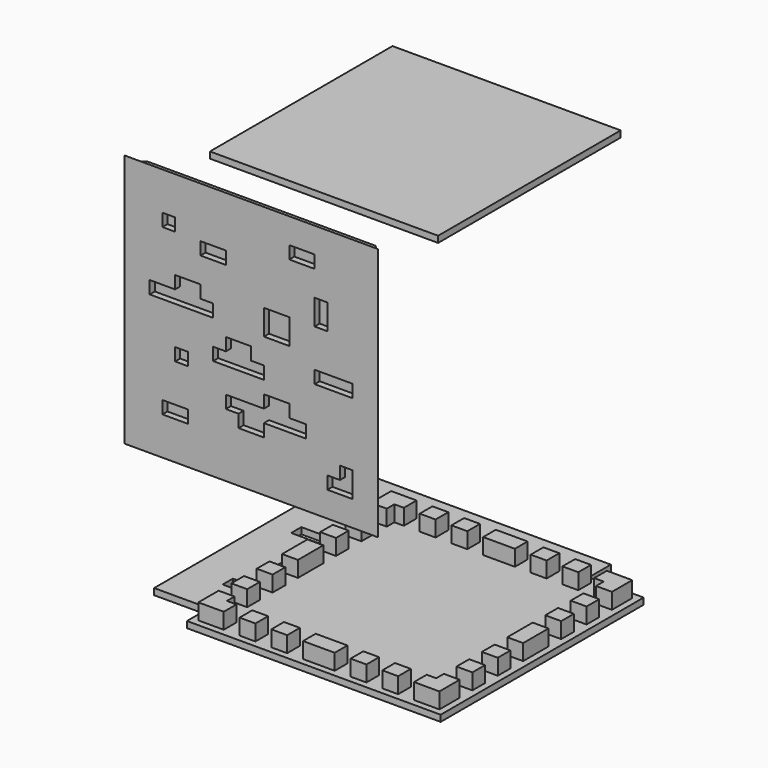
from build123d import *

# Parameters (mm, degrees)
F0_W      = 80
F0_H      = 80
F0_W_2    = 8
F0_H_2    = 4
F0_W_3    = 4
F0_W_4    = 12
F0_H_3    = 8
F1_DEPTH  = 2
F2_W      = 80
F2_H      = 80
F3_DEPTH  = 2
F4_W      = 76
F4_H      = 76
F4_W_2    = 66
F4_H_2    = 66
F5_DEPTH  = 5
F6_W      = 5
F6_H      = 5
F7_DEPTH  = 5
F8_W      = 80
F8_H      = 80
F8_W_2    = 8
F8_H_2    = 4
F8_W_3    = 4
F8_W_4    = 12
F8_H_3    = 8
F9_DEPTH  = 2
F13_DEPTH = 80
F15_DEPTH = 80
F17_DEPTH = 5
F18_W     = 12
F18_H     = 4
F18_W_2   = 8
F18_W_3   = 4
F18_H_2   = 8
F18_W_4   = 1.9
F18_H_3   = 2.2186623164
F19_DEPTH = 2
F21_DEPTH = 73
F22_DEPTH = 5
F24_W     = 71.95
F24_H     = 71.95
F25_DEPTH = 2


with BuildPart() as f1:
    # F0 (on Top) → F1 (new body)
    with BuildSketch(Plane.XY):
        with Locations((-17.2806037962, 8.6768372357)):
            Rectangle(F0_W, F0_H)
        with Locations((-41.2806037962, -17.3231627643)):
            Rectangle(F0_W_2, F0_H_2, mode=Mode.SUBTRACT)
        with Locations((-39.2806037962, -1.3231627643)):
            Rectangle(F0_W_3, F0_H_2, mode=Mode.SUBTRACT)
        Polygon((-25.2806037962, 4.6768372357), (-25.2806037962, 8.6768372357), (-17.2806037962, 8.6768372357), (-17.2806037962, 4.6768372357), (-13.2806037962, 4.6768372357), (-13.2806037962, 0.6768372357), (-29.2806037962, 0.6768372357), (-29.2806037962, 4.6768372357), align=None, mode=Mode.SUBTRACT)
        Polygon((14.7193962038, -23.3231627643), (6.7193962038, -23.3231627643), (6.7193962038, -19.3231627643), (10.7193962038, -19.3231627643), (10.7193962038, -15.3231627643), (14.7193962038, -15.3231627643), (14.7193962038, -19.3231627643), align=None, mode=Mode.SUBTRACT)
        Polygon((-13.2806037962, -7.3231627643), (-13.2806037962, -3.3231627643), (-5.2806037962, -3.3231627643), (-5.2806037962, -7.3231627643), (0, -7.3231627643), (0, -11.3231627643), (-13.2806037962, -11.3231627643), (-13.2806037962, -15.3231627643), (-21.2806037962, -15.3231627643), (-21.2806037962, -11.3231627643), (-25.2806037962, -11.3231627643), (-25.2806037962, -7.3231627643), align=None, mode=Mode.SUBTRACT)
        with Locations((8.7193962038, 6.6768372357)):
            Rectangle(F0_W_4, F0_H_2, mode=Mode.SUBTRACT)
        Polygon((-41.2806037962, 16.6768372357), (-41.2806037962, 20.6768372357), (-33.2806037962, 20.6768372357), (-33.2806037962, 16.6768372357), (-29.2806037962, 16.6768372357), (-29.2806037962, 12.6768372357), (-49.2806037962, 12.6768372357), (-49.2806037962, 16.6768372357), align=None, mode=Mode.SUBTRACT)
        with Locations((-43.2806037962, 34.6768372357)):
            Rectangle(F0_W_3, F0_H_2, mode=Mode.SUBTRACT)
        with Locations((-29.2806037962, 30.6768372357)):
            Rectangle(F0_W_2, F0_H_2, mode=Mode.SUBTRACT)
        with Locations((-9.2806037962, 16.6768372357)):
            Rectangle(F0_W_2, F0_H_3, mode=Mode.SUBTRACT)
        with Locations((4.7193962038, 24.6768372357)):
            Rectangle(F0_W_3, F0_H_3, mode=Mode.SUBTRACT)
        with Locations((-1.2806037962, 38.6768372357)):
            Rectangle(F0_W_2, F0_H_2, mode=Mode.SUBTRACT)
    extrude(amount=F1_DEPTH)


with BuildPart() as f3:
    # F2 (on Top) → F3 (new body)
    with BuildSketch(Plane.XY):
        Rectangle(F2_W, F2_H)
    extrude(amount=F3_DEPTH)

    # F4 (on face) → F5 (join)
    with BuildSketch(Plane.XY.offset(2)):
        Rectangle(F4_W, F4_H)
        Rectangle(F4_W_2, F4_H_2, mode=Mode.SUBTRACT)
    extrude(amount=F5_DEPTH)

    # F6 (on face) → F7 (cut)
    with BuildSketch(Plane.XY.offset(7)):
        with Locations((-35.5, -27.5)):
            Rectangle(F6_W, F6_H)
        with Locations((-35.5, -17.5)):
            Rectangle(F6_W, F6_H)
        with Locations((-35.5, -7.5)):
            Rectangle(F6_W, F6_H)
        with Locations((-35.5, 27.5)):
            Rectangle(F6_W, F6_H)
        with Locations((-35.5, 17.5)):
            Rectangle(F6_W, F6_H)
        with Locations((-35.5, 7.5)):
            Rectangle(F6_W, F6_H)
        with Locations((35.5, -27.5)):
            Rectangle(F6_W, F6_H)
        with Locations((35.5, -17.5)):
            Rectangle(F6_W, F6_H)
        with Locations((35.5, -7.5)):
            Rectangle(F6_W, F6_H)
        with Locations((35.5, 27.5)):
            Rectangle(F6_W, F6_H)
        with Locations((35.5, 17.5)):
            Rectangle(F6_W, F6_H)
        with Locations((35.5, 7.5)):
            Rectangle(F6_W, F6_H)
        with Locations((-27.5, 35.5)):
            Rectangle(F6_W, F6_H)
        with Locations((-17.5, 35.5)):
            Rectangle(F6_W, F6_H)
        with Locations((27.5, 35.5)):
            Rectangle(F6_W, F6_H)
        with Locations((17.5, 35.5)):
            Rectangle(F6_W, F6_H)
        with Locations((7.5, 35.5)):
            Rectangle(F6_W, F6_H)
        with Locations((-7.5, 35.5)):
            Rectangle(F6_W, F6_H)
        with Locations((-27.5, -35.5)):
            Rectangle(F6_W, F6_H)
        with Locations((-17.5, -35.5)):
            Rectangle(F6_W, F6_H)
        with Locations((-7.5, -35.5)):
            Rectangle(F6_W, F6_H)
        with Locations((27.5, -35.5)):
            Rectangle(F6_W, F6_H)
        with Locations((17.5, -35.5)):
            Rectangle(F6_W, F6_H)
        with Locations((7.5, -35.5)):
            Rectangle(F6_W, F6_H)
    extrude(amount=-F7_DEPTH, mode=Mode.SUBTRACT)


with BuildPart() as f9:
    # F8 (on Front) → F9 (new body)
    with BuildSketch(Plane.XZ):
        with Locations((-50.1320821094, 59.4921786048)):
            Rectangle(F8_W, F8_H)
        with Locations((-74.1320821094, 33.4921786048)):
            Rectangle(F8_W_2, F8_H_2, mode=Mode.SUBTRACT)
        with Locations((-72.1320821094, 49.4921786048)):
            Rectangle(F8_W_3, F8_H_2, mode=Mode.SUBTRACT)
        Polygon((-58.1320821094, 55.4921786048), (-58.1320821094, 59.4921786048), (-50.1320821094, 59.4921786048), (-50.1320821094, 55.4921786048), (-46.1320821094, 55.4921786048), (-46.1320821094, 51.4921786048), (-62.1320821094, 51.4921786048), (-62.1320821094, 55.4921786048), align=None, mode=Mode.SUBTRACT)
        Polygon((-18.1320821094, 27.4921786048), (-26.1320821094, 27.4921786048), (-26.1320821094, 31.4921786048), (-22.1320821094, 31.4921786048), (-22.1320821094, 35.4921786048), (-18.1320821094, 35.4921786048), (-18.1320821094, 31.4921786048), align=None, mode=Mode.SUBTRACT)
        Polygon((-46.1320821094, 43.4921786048), (-46.1320821094, 47.4921786048), (-38.1320821094, 47.4921786048), (-38.1320821094, 43.4921786048), (-32.8514783131, 43.4921786048), (-32.8514783131, 39.4921786048), (-46.1320821094, 39.4921786048), (-46.1320821094, 35.4921786048), (-54.1320821094, 35.4921786048), (-54.1320821094, 39.4921786048), (-58.1320821094, 39.4921786048), (-58.1320821094, 43.4921786048), align=None, mode=Mode.SUBTRACT)
        with Locations((-24.1320821094, 57.4921786048)):
            Rectangle(F8_W_4, F8_H_2, mode=Mode.SUBTRACT)
        Polygon((-74.1320821094, 67.4921786048), (-74.1320821094, 71.4921786048), (-66.1320821094, 71.4921786048), (-66.1320821094, 67.4921786048), (-62.1320821094, 67.4921786048), (-62.1320821094, 63.4921786048), (-82.1320821094, 63.4921786048), (-82.1320821094, 67.4921786048), align=None, mode=Mode.SUBTRACT)
        with Locations((-76.1320821094, 85.4921786048)):
            Rectangle(F8_W_3, F8_H_2, mode=Mode.SUBTRACT)
        with Locations((-62.1320821094, 81.4921786048)):
            Rectangle(F8_W_2, F8_H_2, mode=Mode.SUBTRACT)
        with Locations((-42.1320821094, 67.4921786048)):
            Rectangle(F8_W_2, F8_H_3, mode=Mode.SUBTRACT)
        with Locations((-28.1320821094, 75.4921786048)):
            Rectangle(F8_W_3, F8_H_3, mode=Mode.SUBTRACT)
        with Locations((-34.1320821094, 89.4921786048)):
            Rectangle(F8_W_2, F8_H_2, mode=Mode.SUBTRACT)
    extrude(amount=F9_DEPTH)

    # F12 (on offset) → F13 (cut, through all)
    with BuildSketch(Plane.YZ.offset(-10.1320821094)):
        Polygon((0, 99.4921786048), (-2, 99.4921786048), (0, 97.4921786048), align=None)
    extrude(amount=-F13_DEPTH, mode=Mode.SUBTRACT)

    # F14 (on offset) → F15 (cut, through all)
    with BuildSketch(Plane.XY.offset(99.4921786048)):
        Polygon((-12.1320821094, 0), (-10.1320821094, -2), (-10.1320821094, 0), align=None)
        Polygon((-90.1320821094, 0), (-90.1320821094, -2), (-88.1320821094, 0), align=None)
    extrude(amount=-F15_DEPTH, mode=Mode.SUBTRACT)

    # F16 (on face) → F17 (join)
    with BuildSketch(Plane(origin=(0, 0, 0), x_dir=(-1, 0, 0), z_dir=(0, 1, 0))):
        Polygon((21.6320821094, 24.4921786048), (20.1820821094, 24.4921786048), (20.1820821094, 19.5921786048), (25.0820821094, 19.5921786048), (25.0820821094, 24.4921786048), (23.6320821094, 24.4921786048), (23.6320821094, 22.1735162884), (21.6320821094, 22.1735162884), align=None)
        Polygon((31.6320821094, 24.4921786048), (30.1820821094, 24.4921786048), (30.1820821094, 19.5921786048), (35.0820821094, 19.5921786048), (35.0820821094, 24.4921786048), (33.6320821094, 24.4921786048), (33.6320821094, 22.1735162884), (31.6320821094, 22.1735162884), align=None)
        Polygon((41.6320821094, 24.4921786048), (40.1820821094, 24.4921786048), (40.1820821094, 19.5921786048), (45.0820821094, 19.5921786048), (45.0820821094, 24.4921786048), (43.6320821094, 24.4921786048), (43.6320821094, 22.1735162884), (41.6320821094, 22.1735162884), align=None)
        Polygon((56.6320821094, 24.4921786048), (55.1820821094, 24.4921786048), (55.1820821094, 19.5921786048), (60.0820821094, 19.5921786048), (60.0820821094, 24.4921786048), (58.6320821094, 24.4921786048), (58.6320821094, 22.1735162884), (56.6320821094, 22.1735162884), align=None)
        Polygon((70.0820821094, 19.5921786048), (70.0820821094, 24.4921786048), (68.6320821094, 24.4921786048), (68.6320821094, 22.1735162884), (66.6320821094, 22.1735162884), (66.6320821094, 24.4921786048), (65.1820821094, 24.4921786048), (65.1820821094, 19.5921786048), align=None)
        Polygon((80.0820821094, 19.5921786048), (80.0820821094, 24.4921786048), (78.6320821094, 24.4921786048), (78.6320821094, 22.1735162884), (76.6320821094, 22.1735162884), (76.6320821094, 24.4921786048), (75.1820821094, 24.4921786048), (75.1820821094, 19.5921786048), align=None)
    extrude(amount=F17_DEPTH)


with BuildPart() as f19:
    # F18 (on face) → F19 (new body)
    with BuildSketch(Plane(origin=(0, 0, 0), x_dir=(-1, 0, 0), z_dir=(0, 1, 0))):
        Polygon((21.6320821094, 24.4921786048), (21.6820821094, 24.4921786048), (23.5820821094, 24.4921786048), (23.6320821094, 24.4921786048), (25.0820821094, 24.4921786048), (26.6820821094, 24.4921786048), (28.5820821094, 24.4921786048), (30.1820821094, 24.4921786048), (31.6320821094, 24.4921786048), (31.6820821094, 24.4921786048), (33.5820821094, 24.4921786048), (33.6320821094, 24.4921786048), (35.0820821094, 24.4921786048), (36.6820821094, 24.4921786048), (38.5820821094, 24.4921786048), (40.1820821094, 24.4921786048), (41.6320821094, 24.4921786048), (41.6820821094, 24.4921786048), (43.5820821094, 24.4921786048), (43.6320821094, 24.4921786048), (45.0820821094, 24.4921786048), (46.6820821094, 24.4921786048), (48.5820821094, 24.4921786048), (51.6820821094, 24.4921786048), (53.5820821094, 24.4921786048), (55.1820821094, 24.4921786048), (56.6320821094, 24.4921786048), (56.6820821094, 24.4921786048), (58.5820821094, 24.4921786048), (58.6320821094, 24.4921786048), (60.0820821094, 24.4921786048), (61.6820821094, 24.4921786048), (63.5820821094, 24.4921786048), (65.1820821094, 24.4921786048), (66.6320821094, 24.4921786048), (66.6820821094, 24.4921786048), (68.5820821094, 24.4921786048), (68.6320821094, 24.4921786048), (70.0820821094, 24.4921786048), (71.6820821094, 24.4921786048), (73.5820821094, 24.4921786048), (75.1820821094, 24.4921786048), (76.6320821094, 24.4921786048), (76.6820821094, 24.4921786048), (78.5820821094, 24.4921786048), (78.6320821094, 24.4921786048), (80.0820821094, 24.4921786048), (88.1320821094, 24.4921786048), (88.1320821094, 97.4921786048), (12.1320821093, 97.4921786048), (12.1320821094, 24.4921786048), (20.1820821094, 24.4921786048), align=None)
        Polygon((26.1320821094, 31.4921786048), (26.1320821094, 27.4921786048), (18.1320821094, 27.4921786048), (18.1320821094, 35.4921786048), (22.1320821094, 35.4921786048), (22.1320821094, 31.4921786048), align=None, mode=Mode.SUBTRACT)
        with Locations((24.1320821094, 57.4921786048)):
            Rectangle(F18_W, F18_H, mode=Mode.SUBTRACT)
        Polygon((38.1320821094, 47.4921786048), (46.1320821094, 47.4921786048), (46.1320821094, 43.4921786048), (58.1320821094, 43.4921786048), (58.1320821094, 39.4921786048), (54.1320821094, 39.4921786048), (54.1320821094, 35.4921786048), (46.1320821094, 35.4921786048), (46.1320821094, 39.4921786048), (32.8514783131, 39.4921786048), (32.8514783131, 43.4921786048), (38.1320821094, 43.4921786048), align=None, mode=Mode.SUBTRACT)
        with Locations((74.1320821094, 33.4921786048)):
            Rectangle(F18_W_2, F18_H, mode=Mode.SUBTRACT)
        Polygon((46.1320821094, 51.4921786048), (46.1320821094, 55.4921786048), (50.1320821094, 55.4921786048), (50.1320821094, 59.4921786048), (58.1320821094, 59.4921786048), (58.1320821094, 55.4921786048), (62.1320821094, 55.4921786048), (62.1320821094, 51.4921786048), align=None, mode=Mode.SUBTRACT)
        with Locations((72.1320821094, 49.4921786048)):
            Rectangle(F18_W_3, F18_H, mode=Mode.SUBTRACT)
        with Locations((28.1320821094, 75.4921786048)):
            Rectangle(F18_W_3, F18_H_2, mode=Mode.SUBTRACT)
        with Locations((42.1320821094, 67.4921786048)):
            Rectangle(F18_W_2, F18_H_2, mode=Mode.SUBTRACT)
        with Locations((34.1320821094, 89.4921786048)):
            Rectangle(F18_W_2, F18_H, mode=Mode.SUBTRACT)
        Polygon((66.1320821094, 71.4921786048), (74.1320821094, 71.4921786048), (74.1320821094, 67.4921786048), (82.1320821094, 67.4921786048), (82.1320821094, 63.4921786048), (62.1320821094, 63.4921786048), (62.1320821094, 67.4921786048), (66.1320821094, 67.4921786048), align=None, mode=Mode.SUBTRACT)
        with Locations((62.1320821094, 81.4921786048)):
            Rectangle(F18_W_2, F18_H, mode=Mode.SUBTRACT)
        with Locations((76.1320821094, 85.4921786048)):
            Rectangle(F18_W_3, F18_H, mode=Mode.SUBTRACT)
        Polygon((46.1320821094, 43.4921786048), (46.1320821094, 47.4921786048), (38.1320821094, 47.4921786048), (38.1320821094, 43.4921786048), (32.8514783131, 43.4921786048), (32.8514783131, 39.4921786048), (46.1320821094, 39.4921786048), (46.1320821094, 35.4921786048), (54.1320821094, 35.4921786048), (54.1320821094, 39.4921786048), (58.1320821094, 39.4921786048), (58.1320821094, 43.4921786048), align=None)
        Polygon((74.1320821094, 67.4921786048), (74.1320821094, 71.4921786048), (66.1320821094, 71.4921786048), (66.1320821094, 67.4921786048), (62.1320821094, 67.4921786048), (62.1320821094, 63.4921786048), (82.1320821094, 63.4921786048), (82.1320821094, 67.4921786048), align=None)
        Polygon((50.1320821094, 55.4921786048), (46.1320821094, 55.4921786048), (46.1320821094, 51.4921786048), (62.1320821094, 51.4921786048), (62.1320821094, 55.4921786048), (58.1320821094, 55.4921786048), (58.1320821094, 59.4921786048), (50.1320821094, 59.4921786048), align=None)
        with Locations((42.1320821094, 67.4921786048)):
            Rectangle(F18_W_2, F18_H_2)
        with Locations((24.1320821094, 57.4921786048)):
            Rectangle(F18_W, F18_H)
        Polygon((18.1320821094, 27.4921786048), (26.1320821094, 27.4921786048), (26.1320821094, 31.4921786048), (22.1320821094, 31.4921786048), (22.1320821094, 35.4921786048), (18.1320821094, 35.4921786048), align=None)
        with Locations((62.1320821094, 81.4921786048)):
            Rectangle(F18_W_2, F18_H)
        with Locations((28.1320821094, 75.4921786048)):
            Rectangle(F18_W_3, F18_H_2)
        with Locations((34.1320821094, 89.4921786048)):
            Rectangle(F18_W_2, F18_H)
        with Locations((74.1320821094, 33.4921786048)):
            Rectangle(F18_W_2, F18_H)
        with Locations((76.1320821094, 85.4921786048)):
            Rectangle(F18_W_3, F18_H)
        with Locations((72.1320821094, 49.4921786048)):
            Rectangle(F18_W_3, F18_H)
        with Locations((42.6320821094, 23.3828474466)):
            Rectangle(F18_W_4, F18_H_3)
        with Locations((67.6320821094, 23.3828474466)):
            Rectangle(F18_W_4, F18_H_3)
        with Locations((77.6320821094, 23.3828474466)):
            Rectangle(F18_W_4, F18_H_3)
        with Locations((32.6320821094, 23.3828474466)):
            Rectangle(F18_W_4, F18_H_3)
        with Locations((57.6320821094, 23.3828474466)):
            Rectangle(F18_W_4, F18_H_3)
        with Locations((22.6320821094, 23.3828474466)):
            Rectangle(F18_W_4, F18_H_3)
    extrude(amount=F19_DEPTH)

    # F20 (on face) → F21 (cut, through all)
    with BuildSketch(Plane.XY.offset(97.4921786048)):
        Polygon((-14.1320821093, 2), (-12.1320821093, 0), (-12.1320821093, 2), align=None)
        Polygon((-88.1320821095, 2), (-88.1320821095, 0), (-86.1320821095, 2), align=None)
    extrude(amount=-F21_DEPTH, mode=Mode.SUBTRACT)

    # F18 (on face) → F22 (join)
    with BuildSketch(Plane(origin=(0, 0, 0), x_dir=(-1, 0, 0), z_dir=(0, 1, 0))):
        with Locations((22.6320821094, 23.3828474466)):
            Rectangle(F18_W_4, F18_H_3)
        Polygon((31.6820821094, 24.4921786048), (31.6320821094, 24.4921786048), (31.6320821094, 22.1735162884), (33.6320821094, 22.1735162884), (33.6320821094, 24.4921786048), (33.5820821094, 24.4921786048), (33.5820821094, 22.2735162884), (31.6820821094, 22.2735162884), align=None)
        with Locations((32.6320821094, 23.3828474466)):
            Rectangle(F18_W_4, F18_H_3)
        with Locations((42.6320821094, 23.3828474466)):
            Rectangle(F18_W_4, F18_H_3)
        with Locations((77.6320821094, 23.3828474466)):
            Rectangle(F18_W_4, F18_H_3)
        with Locations((67.6320821094, 23.3828474466)):
            Rectangle(F18_W_4, F18_H_3)
        with Locations((57.6320821094, 23.3828474466)):
            Rectangle(F18_W_4, F18_H_3)
    extrude(amount=F22_DEPTH)


with BuildPart() as f25:
    # F24 (on offset) → F25 (new body)
    with BuildSketch(Plane.XY.offset(130)):
        Rectangle(F24_W, F24_H)
    extrude(amount=F25_DEPTH)


solid = Compound([f1.part, f3.part, f9.part, f19.part, f25.part])
